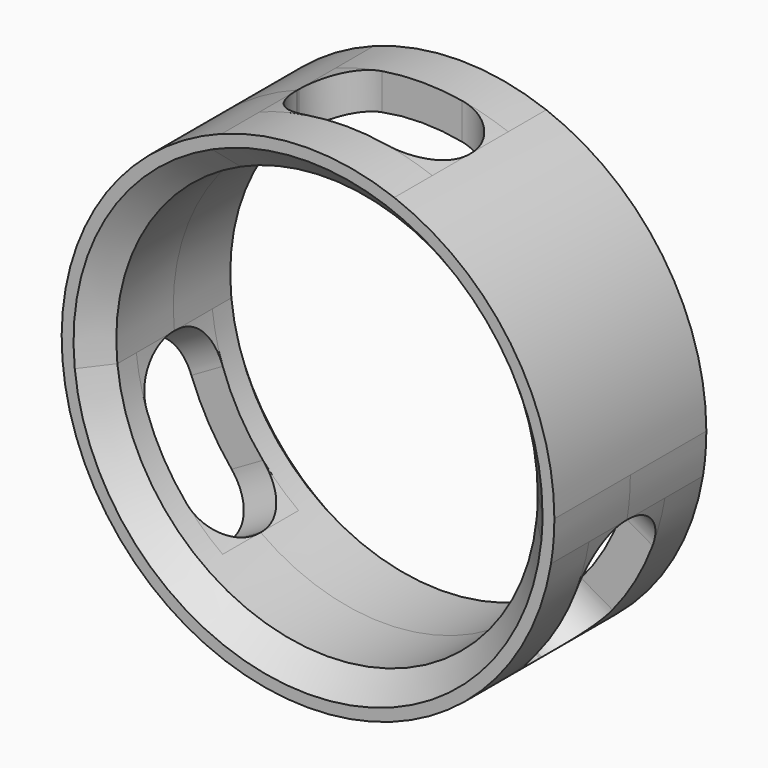
from build123d import *

# Parameters (mm, degrees)
F1_DEPTH      = 4
F1_DEPTH_BACK = 4
F2_SIZE       = 1
F4_DEPTH      = 2
F4_DEPTH_BACK = 2
F5_T4_DEPTH   = 11.3208024162
F5_S5_R       = 8.875
F5_T6_DEPTH   = 8
F5_S7_R       = 10.375
F5_T8_DEPTH   = 8
F5_T12_DEPTH  = 11.3208024162
F5_S13_R      = 10.375
F5_T14_DEPTH  = 8
F5_S15_R      = 8.875
F5_T16_DEPTH  = 8
F5_T20_DEPTH  = 11.3208024162
F5_S21_R      = 8.875
F5_T22_DEPTH  = 8
F5_S23_R      = 10.375
F5_T24_DEPTH  = 8
F5_T28_DEPTH  = 11.3208024162
F5_S29_R      = 8.875
F5_T30_DEPTH  = 8
F5_S31_R      = 10.375
F5_T32_DEPTH  = 8
F5_T36_DEPTH  = 11.3208024162
F5_S37_R      = 8.875
F5_T38_DEPTH  = 8
F5_S39_R      = 10.375
F5_T40_DEPTH  = 8
F5_T44_DEPTH  = 11.3208024162
F5_S45_R      = 8.875
F5_T46_DEPTH  = 8
F5_S47_R      = 10.375
F5_T48_DEPTH  = 8
F5_T52_DEPTH  = 11.3208024162
F5_S53_R      = 8.875
F5_T54_DEPTH  = 8
F5_S55_R      = 10.375
F5_T56_DEPTH  = 8
F5_T60_DEPTH  = 11.3208024162
F5_S61_R      = 8.875
F5_T62_DEPTH  = 8
F5_S63_R      = 10.375
F5_T64_DEPTH  = 8
F5_T68_DEPTH  = 11.3208024162
F5_S69_R      = 8.875
F5_T70_DEPTH  = 7
F5_S71_R      = 10.375
F5_T72_DEPTH  = 7
F5_T76_DEPTH  = 11.3208024162
F5_S77_R      = 8.875
F5_T78_DEPTH  = 7
F5_S79_R      = 10.375
F5_T80_DEPTH  = 7
F5_T84_DEPTH  = 11.3208024162
F5_S85_R      = 8.875
F5_T86_DEPTH  = 7
F5_S87_R      = 10.375
F5_T88_DEPTH  = 7
F5_T92_DEPTH  = 11.3208024162
F5_S93_R      = 8.875
F5_T94_DEPTH  = 7
F5_S95_R      = 10.375
F5_T96_DEPTH  = 7


# Not quite as in the source:
# - a fillet or chamfer that OpenCascade refuses, or shapes differently, is made with other operations: its cross-section is extruded or revolved along the edge and cut away or added


with BuildPart() as f1:
    # F0 (on Front) → F1 (new body, two sides)
    with BuildSketch(Plane.XZ) as f1_sk:
        with BuildLine():
            ThreePointArc((-3.6332620451, 8.0972237163), (0, 8.875), (3.6332620451, 8.0972237163))
            Line((3.6332620451, 8.0972237163), (3.6332620451, 9.7180261325))
            ThreePointArc((3.6332620451, 9.7180261325), (0, 10.375), (-3.6332620451, 9.7180261325))
            Line((-3.6332620451, 9.7180261325), (-3.6332620451, 8.0972237163))
        make_face()
        with BuildLine():
            ThreePointArc((-8.829032461, -0.9021146285), (-7.6859754586, 4.4375), (-3.6332620451, 8.0972237163))
            Line((-3.6332620451, 8.0972237163), (-3.6332620451, 9.7180261325))
            ThreePointArc((-3.6332620451, 9.7180261325), (-8.9850135643, 5.1875), (-10.2326885279, -1.7125158366))
            Line((-10.2326885279, -1.7125158366), (-8.829032461, -0.9021146285))
        make_face()
        with BuildLine():
            ThreePointArc((-5.1957704159, -7.1951090878), (-7.6859754586, -4.4375), (-8.829032461, -0.9021146285))
            Line((-8.829032461, -0.9021146285), (-10.2326885279, -1.7125158366))
            ThreePointArc((-10.2326885279, -1.7125158366), (-8.9850135643, -5.1875), (-6.5994264829, -8.0055102959))
            Line((-6.5994264829, -8.0055102959), (-5.1957704159, -7.1951090878))
        make_face()
        with BuildLine():
            Line((6.5994264829, -8.0055102959), (5.1957704159, -7.1951090878))
            ThreePointArc((5.1957704159, -7.1951090878), (0, -8.875), (-5.1957704159, -7.1951090878))
            Line((-5.1957704159, -7.1951090878), (-6.5994264829, -8.0055102959))
            ThreePointArc((-6.5994264829, -8.0055102959), (0, -10.375), (6.5994264829, -8.0055102959))
        make_face()
        with BuildLine():
            Line((10.2326885279, -1.7125158366), (8.829032461, -0.9021146285))
            ThreePointArc((8.829032461, -0.9021146285), (7.6859754586, -4.4375), (5.1957704159, -7.1951090878))
            Line((5.1957704159, -7.1951090878), (6.5994264829, -8.0055102959))
            ThreePointArc((6.5994264829, -8.0055102959), (8.9850135643, -5.1875), (10.2326885279, -1.7125158366))
        make_face()
        with BuildLine():
            ThreePointArc((3.6332620451, 8.0972237163), (7.450195489, 4.8228842175), (8.875, 0))
            ThreePointArc((8.875, 0), (8.8635006654, -0.4516425073), (8.829032461, -0.9021146285))
            Line((8.829032461, -0.9021146285), (10.2326885279, -1.7125158366))
            ThreePointArc((10.2326885279, -1.7125158366), (10.3393609202, -0.8592093816), (10.375, 0))
            ThreePointArc((10.375, 0), (8.524544525, 5.9137776118), (3.6332620451, 9.7180261325))
            Line((3.6332620451, 9.7180261325), (3.6332620451, 8.0972237163))
        make_face()
        with BuildLine():
            ThreePointArc((-5.1957704159, -7.1951090878), (-7.6859754586, -4.4375), (-8.829032461, -0.9021146285))
            Line((-8.829032461, -0.9021146285), (-10.2326885279, -1.7125158366))
            ThreePointArc((-10.2326885279, -1.7125158366), (-8.9850135643, -5.1875), (-6.5994264829, -8.0055102959))
            Line((-6.5994264829, -8.0055102959), (-5.1957704159, -7.1951090878))
        make_face()
        with BuildLine():
            ThreePointArc((3.6332620451, 8.0972237163), (7.450195489, 4.8228842175), (8.875, 0))
            ThreePointArc((8.875, 0), (8.8635006654, -0.4516425073), (8.829032461, -0.9021146285))
            Line((8.829032461, -0.9021146285), (10.2326885279, -1.7125158366))
            ThreePointArc((10.2326885279, -1.7125158366), (10.3393609202, -0.8592093816), (10.375, 0))
            ThreePointArc((10.375, 0), (8.524544525, 5.9137776118), (3.6332620451, 9.7180261325))
            Line((3.6332620451, 9.7180261325), (3.6332620451, 8.0972237163))
        make_face()
        with BuildLine():
            ThreePointArc((-8.829032461, -0.9021146285), (-7.6859754586, 4.4375), (-3.6332620451, 8.0972237163))
            Line((-3.6332620451, 8.0972237163), (-3.6332620451, 9.7180261325))
            ThreePointArc((-3.6332620451, 9.7180261325), (-8.9850135643, 5.1875), (-10.2326885279, -1.7125158366))
            Line((-10.2326885279, -1.7125158366), (-8.829032461, -0.9021146285))
        make_face()
        with BuildLine():
            ThreePointArc((-5.1957704159, -7.1951090878), (-7.6859754586, -4.4375), (-8.829032461, -0.9021146285))
            Line((-8.829032461, -0.9021146285), (-10.2326885279, -1.7125158366))
            ThreePointArc((-10.2326885279, -1.7125158366), (-8.9850135643, -5.1875), (-6.5994264829, -8.0055102959))
            Line((-6.5994264829, -8.0055102959), (-5.1957704159, -7.1951090878))
        make_face()
    extrude(amount=F1_DEPTH)
    extrude(f1_sk.sketch, amount=-F1_DEPTH_BACK)

    # F2
    f2_edges = [f1.edges().sort_by_distance(p)[0] for p in [
        (-8.829032, -4, 0.902115),
        (-8.829032, 4, 0.902115),
    ]]
    chamfer(f2_edges, length=F2_SIZE)

    # F0 (on Front) → F4 (cut, two sides)
    with BuildSketch(Plane.XZ) as f4_sk:
        with BuildLine():
            ThreePointArc((-3.6332620451, 9.7180261325), (0, 10.375), (3.6332620451, 9.7180261325))
            Line((3.6332620451, 9.7180261325), (3.6332620451, 11.8753320796))
            Line((3.6332620451, 11.8753320796), (-3.6332620451, 11.8753320796))
            Line((-3.6332620451, 11.8753320796), (-3.6332620451, 9.7180261325))
        make_face()
        with BuildLine():
            ThreePointArc((-3.6332620451, 8.0972237163), (0, 8.875), (3.6332620451, 8.0972237163))
            Line((3.6332620451, 8.0972237163), (3.6332620451, 9.7180261325))
            ThreePointArc((3.6332620451, 9.7180261325), (0, 10.375), (-3.6332620451, 9.7180261325))
            Line((-3.6332620451, 9.7180261325), (-3.6332620451, 8.0972237163))
        make_face()
        with BuildLine():
            Line((3.6332620451, 6.6060326062), (3.6332620451, 8.0972237163))
            ThreePointArc((3.6332620451, 8.0972237163), (0, 8.875), (-3.6332620451, 8.0972237163))
            Line((-3.6332620451, 8.0972237163), (-3.6332620451, 6.6060326062))
            Line((-3.6332620451, 6.6060326062), (3.6332620451, 6.6060326062))
        make_face()
        with BuildLine():
            ThreePointArc((5.1957704159, -7.1951090878), (7.6859754586, -4.4375), (8.829032461, -0.9021146285))
            Line((8.829032461, -0.9021146285), (7.2665240901, 0))
            Line((7.2665240901, 0), (3.3491878185, -6.1289841281))
            Line((3.3491878185, -6.1289841281), (5.1957704159, -7.1951090878))
        make_face()
        with BuildLine():
            Line((10.2326885279, -1.7125158366), (8.829032461, -0.9021146285))
            ThreePointArc((8.829032461, -0.9021146285), (7.6859754586, -4.4375), (5.1957704159, -7.1951090878))
            Line((5.1957704159, -7.1951090878), (6.5994264829, -8.0055102959))
            ThreePointArc((6.5994264829, -8.0055102959), (8.9850135643, -5.1875), (10.2326885279, -1.7125158366))
        make_face()
        with BuildLine():
            Line((12.1009702818, -2.7911688102), (10.2326885279, -1.7125158366))
            ThreePointArc((10.2326885279, -1.7125158366), (8.9850135643, -5.1875), (6.5994264829, -8.0055102959))
            Line((6.5994264829, -8.0055102959), (8.4677082368, -9.0841632694))
            Line((8.4677082368, -9.0841632694), (12.1009702818, -2.7911688102))
        make_face()
        with BuildLine():
            Line((-6.8559292529, 0.2370570398), (-8.829032461, -0.9021146285))
            ThreePointArc((-8.829032461, -0.9021146285), (-7.6859754586, -4.4375), (-5.1957704159, -7.1951090878))
            Line((-5.1957704159, -7.1951090878), (-3.2841431884, -6.0914305934))
            Line((-3.2841431884, -6.0914305934), (-6.8559292529, 0.2370570398))
        make_face()
        with BuildLine():
            ThreePointArc((-6.5994264829, -8.0055102959), (-8.9850135643, -5.1875), (-10.2326885279, -1.7125158366))
            Line((-10.2326885279, -1.7125158366), (-12.1009702818, -2.7911688102))
            Line((-12.1009702818, -2.7911688102), (-8.4677082368, -9.0841632694))
            Line((-8.4677082368, -9.0841632694), (-6.5994264829, -8.0055102959))
        make_face()
        with BuildLine():
            ThreePointArc((-5.1957704159, -7.1951090878), (-7.6859754586, -4.4375), (-8.829032461, -0.9021146285))
            Line((-8.829032461, -0.9021146285), (-10.2326885279, -1.7125158366))
            ThreePointArc((-10.2326885279, -1.7125158366), (-8.9850135643, -5.1875), (-6.5994264829, -8.0055102959))
            Line((-6.5994264829, -8.0055102959), (-5.1957704159, -7.1951090878))
        make_face()
    extrude(amount=-F4_DEPTH, mode=Mode.SUBTRACT)
    extrude(f4_sk.sketch, amount=F4_DEPTH_BACK, mode=Mode.SUBTRACT)

    # F5: fillet of radius 1.94 on 12 edges, made by hand


with BuildPart() as f5_tool2:
    # F5_s3 → F5_t4 (new body)
    with BuildSketch(Plane(origin=(2.8121782301, 0, -1.6236118582), x_dir=(0, 1, 0), z_dir=(0.8660254038, 0, -0.5))):
        with BuildLine():
            ThreePointArc((0.06, -3.6332620451), (1.4317871555, -3.0650492006), (2, -1.6932620451))
            Line((2, -1.6932620451), (2, -3.6332620451))
            Line((2, -3.6332620451), (0.06, -3.6332620451))
        make_face()
    extrude(amount=F5_T4_DEPTH)

    # F5_s5 → F5_t6 (cut, symmetric)
    with BuildSketch(Plane.XZ.offset(-1)):
        Circle(F5_S5_R)
    extrude(amount=F5_T6_DEPTH, both=True, mode=Mode.SUBTRACT)

    # F5_s7 → F5_t8 (intersect, symmetric)
    with BuildSketch(Plane.XZ.offset(-1)):
        Circle(F5_S7_R)
    extrude(amount=F5_T8_DEPTH, both=True, mode=Mode.INTERSECT)


with BuildPart() as f1_1:
    add(f1.part)

    # F5_t1: union F5_tool2
    add(f5_tool2.part)


with BuildPart() as f5_tool10:
    # F5_s11 → F5_t12 (new body)
    with BuildSketch(Plane(origin=(12.6162807137, 0, -7.2840130663), x_dir=(0, 1, 0), z_dir=(-0.8660254038, 0, 0.5))):
        with BuildLine():
            ThreePointArc((0.06, -3.6332620451), (1.4317871555, -3.0650492006), (2, -1.6932620451))
            Line((2, -1.6932620451), (2, -3.6332620451))
            Line((2, -3.6332620451), (0.06, -3.6332620451))
        make_face()
    extrude(amount=F5_T12_DEPTH)

    # F5_s13 → F5_t14 (intersect, symmetric)
    with BuildSketch(Plane.XZ.offset(-1)):
        Circle(F5_S13_R)
    extrude(amount=F5_T14_DEPTH, both=True, mode=Mode.INTERSECT)

    # F5_s15 → F5_t16 (cut, symmetric)
    with BuildSketch(Plane.XZ.offset(-1)):
        Circle(F5_S15_R)
    extrude(amount=F5_T16_DEPTH, both=True, mode=Mode.SUBTRACT)


with BuildPart() as f1_2:
    add(f1_1.part)

    # F5_t9: union F5_tool10
    add(f5_tool10.part)


with BuildPart() as f5_tool18:
    # F5_s19 → F5_t20 (new body)
    with BuildSketch(Plane(origin=(12.6162807137, 0, -7.2840130663), x_dir=(0, 1, 0), z_dir=(-0.8660254038, 0, 0.5))):
        with BuildLine():
            ThreePointArc((-0.06, -3.6332620451), (-1.4317871555, -3.0650492006), (-2, -1.6932620451))
            Line((-2, -1.6932620451), (-2, -3.6332620451))
            Line((-2, -3.6332620451), (-0.06, -3.6332620451))
        make_face()
    extrude(amount=F5_T20_DEPTH)

    # F5_s21 → F5_t22 (cut, symmetric)
    with BuildSketch(Plane.XZ.offset(1)):
        Circle(F5_S21_R)
    extrude(amount=F5_T22_DEPTH, both=True, mode=Mode.SUBTRACT)

    # F5_s23 → F5_t24 (intersect, symmetric)
    with BuildSketch(Plane.XZ.offset(1)):
        Circle(F5_S23_R)
    extrude(amount=F5_T24_DEPTH, both=True, mode=Mode.INTERSECT)


with BuildPart() as f1_3:
    add(f1_2.part)

    # F5_t17: union F5_tool18
    add(f5_tool18.part)


with BuildPart() as f5_tool26:
    # F5_s27 → F5_t28 (new body)
    with BuildSketch(Plane(origin=(2.8121782301, 0, -1.6236118582), x_dir=(0, 1, 0), z_dir=(0.8660254038, 0, -0.5))):
        with BuildLine():
            ThreePointArc((-2, -1.6932620451), (-1.4317871555, -3.0650492006), (-0.06, -3.6332620451))
            Line((-0.06, -3.6332620451), (-2, -3.6332620451))
            Line((-2, -3.6332620451), (-2, -1.6932620451))
        make_face()
    extrude(amount=F5_T28_DEPTH)

    # F5_s29 → F5_t30 (cut, symmetric)
    with BuildSketch(Plane.XZ.offset(1)):
        Circle(F5_S29_R)
    extrude(amount=F5_T30_DEPTH, both=True, mode=Mode.SUBTRACT)

    # F5_s31 → F5_t32 (intersect, symmetric)
    with BuildSketch(Plane.XZ.offset(1)):
        Circle(F5_S31_R)
    extrude(amount=F5_T32_DEPTH, both=True, mode=Mode.INTERSECT)


with BuildPart() as f1_4:
    add(f1_3.part)

    # F5_t25: union F5_tool26
    add(f5_tool26.part)


with BuildPart() as f5_tool34:
    # F5_s35 → F5_t36 (new body)
    with BuildSketch(Plane(origin=(-12.6162807137, 0, -7.2840130663), x_dir=(0, 1, 0), z_dir=(0.8660254038, 0, 0.5))):
        with BuildLine():
            ThreePointArc((0.06, -3.6332620451), (1.4317871555, -3.0650492006), (2, -1.6932620451))
            Line((2, -1.6932620451), (2, -3.6332620451))
            Line((2, -3.6332620451), (0.06, -3.6332620451))
        make_face()
    extrude(amount=F5_T36_DEPTH)

    # F5_s37 → F5_t38 (cut, symmetric)
    with BuildSketch(Plane.XZ.offset(-1)):
        Circle(F5_S37_R)
    extrude(amount=F5_T38_DEPTH, both=True, mode=Mode.SUBTRACT)

    # F5_s39 → F5_t40 (intersect, symmetric)
    with BuildSketch(Plane.XZ.offset(-1)):
        Circle(F5_S39_R)
    extrude(amount=F5_T40_DEPTH, both=True, mode=Mode.INTERSECT)


with BuildPart() as f1_5:
    add(f1_4.part)

    # F5_t33: union F5_tool34
    add(f5_tool34.part)


with BuildPart() as f5_tool42:
    # F5_s43 → F5_t44 (new body)
    with BuildSketch(Plane(origin=(-2.8121782301, 0, -1.6236118582), x_dir=(0, 1, 0), z_dir=(-0.8660254038, 0, -0.5))):
        with BuildLine():
            ThreePointArc((0.06, -3.6332620451), (1.4317871555, -3.0650492006), (2, -1.6932620451))
            Line((2, -1.6932620451), (2, -3.6332620451))
            Line((2, -3.6332620451), (0.06, -3.6332620451))
        make_face()
    extrude(amount=F5_T44_DEPTH)

    # F5_s45 → F5_t46 (cut, symmetric)
    with BuildSketch(Plane.XZ.offset(-1)):
        Circle(F5_S45_R)
    extrude(amount=F5_T46_DEPTH, both=True, mode=Mode.SUBTRACT)

    # F5_s47 → F5_t48 (intersect, symmetric)
    with BuildSketch(Plane.XZ.offset(-1)):
        Circle(F5_S47_R)
    extrude(amount=F5_T48_DEPTH, both=True, mode=Mode.INTERSECT)


with BuildPart() as f1_6:
    add(f1_5.part)

    # F5_t41: union F5_tool42
    add(f5_tool42.part)


with BuildPart() as f5_tool50:
    # F5_s51 → F5_t52 (new body)
    with BuildSketch(Plane(origin=(-2.8121782301, 0, -1.6236118582), x_dir=(0, 1, 0), z_dir=(-0.8660254038, 0, -0.5))):
        with BuildLine():
            ThreePointArc((-2, -1.6932620451), (-1.4317871555, -3.0650492006), (-0.06, -3.6332620451))
            Line((-0.06, -3.6332620451), (-2, -3.6332620451))
            Line((-2, -3.6332620451), (-2, -1.6932620451))
        make_face()
    extrude(amount=F5_T52_DEPTH)

    # F5_s53 → F5_t54 (cut, symmetric)
    with BuildSketch(Plane.XZ.offset(1)):
        Circle(F5_S53_R)
    extrude(amount=F5_T54_DEPTH, both=True, mode=Mode.SUBTRACT)

    # F5_s55 → F5_t56 (intersect, symmetric)
    with BuildSketch(Plane.XZ.offset(1)):
        Circle(F5_S55_R)
    extrude(amount=F5_T56_DEPTH, both=True, mode=Mode.INTERSECT)


with BuildPart() as f1_7:
    add(f1_6.part)

    # F5_t49: union F5_tool50
    add(f5_tool50.part)


with BuildPart() as f5_tool58:
    # F5_s59 → F5_t60 (new body)
    with BuildSketch(Plane(origin=(-12.6162807137, 0, -7.2840130663), x_dir=(0, 1, 0), z_dir=(0.8660254038, 0, 0.5))):
        with BuildLine():
            ThreePointArc((-0.06, -3.6332620451), (-1.4317871555, -3.0650492006), (-2, -1.6932620451))
            Line((-2, -1.6932620451), (-2, -3.6332620451))
            Line((-2, -3.6332620451), (-0.06, -3.6332620451))
        make_face()
    extrude(amount=F5_T60_DEPTH)

    # F5_s61 → F5_t62 (cut, symmetric)
    with BuildSketch(Plane.XZ.offset(1)):
        Circle(F5_S61_R)
    extrude(amount=F5_T62_DEPTH, both=True, mode=Mode.SUBTRACT)

    # F5_s63 → F5_t64 (intersect, symmetric)
    with BuildSketch(Plane.XZ.offset(1)):
        Circle(F5_S63_R)
    extrude(amount=F5_T64_DEPTH, both=True, mode=Mode.INTERSECT)


with BuildPart() as f1_8:
    add(f1_7.part)

    # F5_t57: union F5_tool58
    add(f5_tool58.part)


with BuildPart() as f5_tool66:
    # F5_s67 → F5_t68 (new body)
    with BuildSketch(Plane.XY.offset(14.5680261325)):
        with BuildLine():
            ThreePointArc((-3.6332620451, 0.06), (-3.0650492006, 1.4317871555), (-1.6932620451, 2))
            Line((-1.6932620451, 2), (-3.6332620451, 2))
            Line((-3.6332620451, 2), (-3.6332620451, 0.06))
        make_face()
    extrude(amount=-F5_T68_DEPTH)

    # F5_s69 → F5_t70 (cut, symmetric)
    with BuildSketch(Plane.XZ.offset(-1)):
        Circle(F5_S69_R)
    extrude(amount=F5_T70_DEPTH, both=True, mode=Mode.SUBTRACT)

    # F5_s71 → F5_t72 (intersect, symmetric)
    with BuildSketch(Plane.XZ.offset(-1)):
        Circle(F5_S71_R)
    extrude(amount=F5_T72_DEPTH, both=True, mode=Mode.INTERSECT)


with BuildPart() as f1_9:
    add(f1_8.part)

    # F5_t65: union F5_tool66
    add(f5_tool66.part)


with BuildPart() as f5_tool74:
    # F5_s75 → F5_t76 (new body)
    with BuildSketch(Plane.XY.offset(3.2472237163)):
        with BuildLine():
            ThreePointArc((3.6332620451, 0.06), (3.0650492006, 1.4317871555), (1.6932620451, 2))
            Line((1.6932620451, 2), (3.6332620451, 2))
            Line((3.6332620451, 2), (3.6332620451, 0.06))
        make_face()
    extrude(amount=F5_T76_DEPTH)

    # F5_s77 → F5_t78 (cut, symmetric)
    with BuildSketch(Plane.XZ.offset(-1)):
        Circle(F5_S77_R)
    extrude(amount=F5_T78_DEPTH, both=True, mode=Mode.SUBTRACT)

    # F5_s79 → F5_t80 (intersect, symmetric)
    with BuildSketch(Plane.XZ.offset(-1)):
        Circle(F5_S79_R)
    extrude(amount=F5_T80_DEPTH, both=True, mode=Mode.INTERSECT)


with BuildPart() as f1_10:
    add(f1_9.part)

    # F5_t73: union F5_tool74
    add(f5_tool74.part)


with BuildPart() as f5_tool82:
    # F5_s83 → F5_t84 (new body)
    with BuildSketch(Plane.XY.offset(14.5680261325)):
        with BuildLine():
            ThreePointArc((-3.6332620451, -0.06), (-3.0650492006, -1.4317871555), (-1.6932620451, -2))
            Line((-1.6932620451, -2), (-3.6332620451, -2))
            Line((-3.6332620451, -2), (-3.6332620451, -0.06))
        make_face()
    extrude(amount=-F5_T84_DEPTH)

    # F5_s85 → F5_t86 (cut, symmetric)
    with BuildSketch(Plane.XZ.offset(1)):
        Circle(F5_S85_R)
    extrude(amount=F5_T86_DEPTH, both=True, mode=Mode.SUBTRACT)

    # F5_s87 → F5_t88 (intersect, symmetric)
    with BuildSketch(Plane.XZ.offset(1)):
        Circle(F5_S87_R)
    extrude(amount=F5_T88_DEPTH, both=True, mode=Mode.INTERSECT)


with BuildPart() as f1_11:
    add(f1_10.part)

    # F5_t81: union F5_tool82
    add(f5_tool82.part)


with BuildPart() as f5_tool90:
    # F5_s91 → F5_t92 (new body)
    with BuildSketch(Plane.XY.offset(3.2472237163)):
        with BuildLine():
            ThreePointArc((1.6932620451, -2), (3.0650492006, -1.4317871555), (3.6332620451, -0.06))
            Line((3.6332620451, -0.06), (3.6332620451, -2))
            Line((3.6332620451, -2), (1.6932620451, -2))
        make_face()
    extrude(amount=F5_T92_DEPTH)

    # F5_s93 → F5_t94 (cut, symmetric)
    with BuildSketch(Plane.XZ.offset(1)):
        Circle(F5_S93_R)
    extrude(amount=F5_T94_DEPTH, both=True, mode=Mode.SUBTRACT)

    # F5_s95 → F5_t96 (intersect, symmetric)
    with BuildSketch(Plane.XZ.offset(1)):
        Circle(F5_S95_R)
    extrude(amount=F5_T96_DEPTH, both=True, mode=Mode.INTERSECT)


with BuildPart() as f1_12:
    add(f1_11.part)

    # F5_t89: union F5_tool90
    add(f5_tool90.part)


solid = f1_12.part
